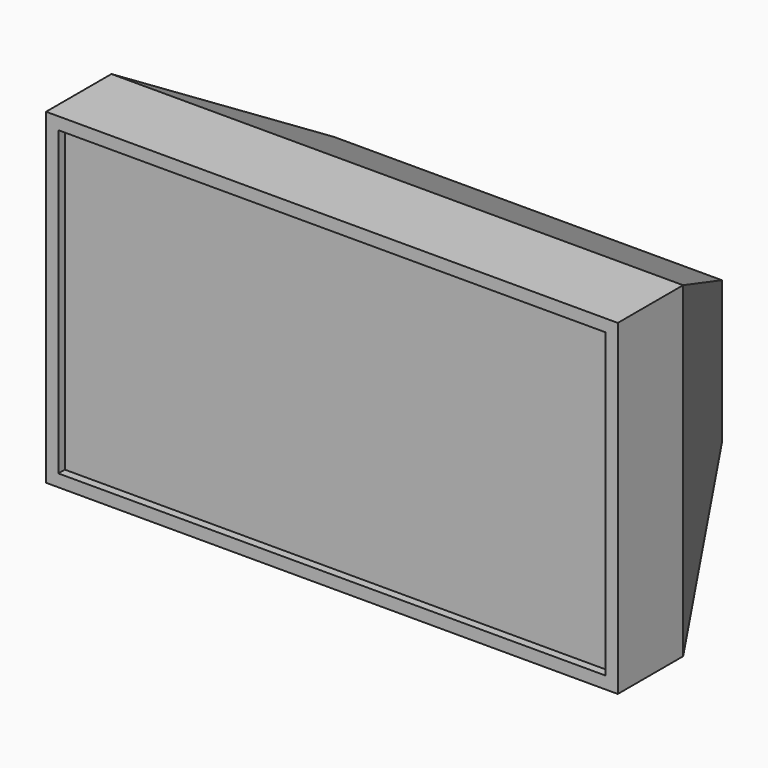
from build123d import *

# Parameters (mm, degrees)
F0_W        = 140
F0_H        = 80
F1_DEPTH    = 60
F2_C1_SIZE2 = 22.5
F2_C1_SIZE  = 40
F2_C2_SIZE2 = 22.5
F2_C2_SIZE  = 40
F2_C3_SIZE2 = 40
F2_C3_SIZE  = 22.5
F2_C4_SIZE2 = 40
F2_C4_SIZE  = 22.5
F3_W        = 134
F3_H        = 74
F4_DEPTH    = 2
F5_DEPTH    = 2


with BuildPart() as f1:
    # F0 (on Front) → F1 (new body)
    with BuildSketch(Plane.XZ):
        Rectangle(F0_W, F0_H)
    extrude(amount=F1_DEPTH)

    # F2: chamfer of 22.5 x 40 on 4 edges, made by hand

    # F2_c1
    f2_c1_edges = [f1.edges().sort_by_distance(p)[0] for p in [
        (0, 0, -40),
    ]]
    f2_c1_side = f1.faces().sort_by_distance((0, -0.45, -40))[0]
    chamfer(f2_c1_edges, length=F2_C1_SIZE, length2=F2_C1_SIZE2, reference=f2_c1_side)

    # F2_c2
    f2_c2_edges = [f1.edges().sort_by_distance(p)[0] for p in [
        (70, 0, 11.25),
    ]]
    f2_c2_side = f1.faces().sort_by_distance((70, -0.45, 11.25))[0]
    chamfer(f2_c2_edges, length=F2_C2_SIZE, length2=F2_C2_SIZE2, reference=f2_c2_side)

    # F2_c3
    f2_c3_edges = [f1.edges().sort_by_distance(p)[0] for p in [
        (-11.25, 0, 40),
    ]]
    f2_c3_side = f1.faces().sort_by_distance((-11.25, 0, 39.55))[0]
    chamfer(f2_c3_edges, length=F2_C3_SIZE, length2=F2_C3_SIZE2, reference=f2_c3_side)

    # F2_c4
    f2_c4_edges = [f1.edges().sort_by_distance(p)[0] for p in [
        (-70, 0, 0),
    ]]
    f2_c4_side = f1.faces().sort_by_distance((-69.55, 0, 0))[0]
    chamfer(f2_c4_edges, length=F2_C4_SIZE, length2=F2_C4_SIZE2, reference=f2_c4_side)

    # F3 (on face) → F4 (join)
    with BuildSketch(Plane.XZ.offset(60)):
        Rectangle(F3_W, F3_H)
    extrude(amount=-F4_DEPTH)

    # F3 (on face) → F5 (cut)
    with BuildSketch(Plane.XZ.offset(60)):
        Rectangle(F3_W, F3_H)
    extrude(amount=-F5_DEPTH, mode=Mode.SUBTRACT)


solid = f1.part
